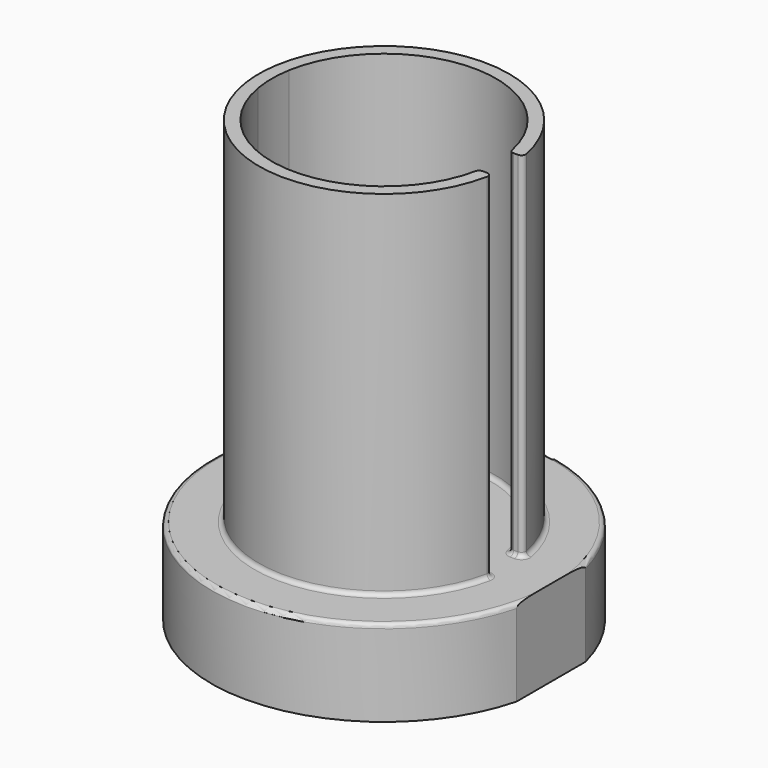
from build123d import *

# Parameters (mm, degrees)
F0_W     = 38.7298334621
F0_H     = 10
F1_DEPTH = 10
F3_DEPTH = 41
F4_F1_R  = 0.5
F4_F2_R  = 0.5


with BuildPart() as f1:
    # F0 (on Top) → F1 (new body)
    with BuildSketch(Plane.XY):
        with BuildLine():
            Line((-19.364916731, 5), (19.364916731, 5))
            ThreePointArc((19.364916731, 5), (0, 20), (-19.364916731, 5))
        make_face()
        Rectangle(F0_W, F0_H)
        with BuildLine():
            ThreePointArc((-19.364916731, -5), (0, -20), (19.364916731, -5))
            Line((19.364916731, -5), (-19.364916731, -5))
        make_face()
        with BuildLine():
            Line((-19.364916731, -5), (-19.364916731, 5))
            ThreePointArc((-19.364916731, 5), (-20, 0), (-19.364916731, -5))
        make_face()
    extrude(amount=-F1_DEPTH)

    # F2 (on face) → F3 (join)
    with BuildSketch(Plane.XY):
        with BuildLine():
            ThreePointArc((-12.8038080273, 2.25), (0, 13), (12.8038080273, 2.25))
            Line((12.8038080273, 2.25), (14.3243673508, 2.25))
            ThreePointArc((14.3243673508, 2.25), (0, 14.5), (-14.3243673508, 2.25))
            Line((-14.3243673508, 2.25), (-12.8038080273, 2.25))
        make_face()
        with BuildLine():
            Line((14.3243673508, -2.25), (12.8038080273, -2.25))
            ThreePointArc((12.8038080273, -2.25), (0, -13), (-12.8038080273, -2.25))
            Line((-12.8038080273, -2.25), (-14.3243673508, -2.25))
            ThreePointArc((-14.3243673508, -2.25), (0, -14.5), (14.3243673508, -2.25))
        make_face()
        with BuildLine():
            ThreePointArc((-12.8038080273, -2.25), (-13, 0), (-12.8038080273, 2.25))
            Line((-12.8038080273, 2.25), (-14.3243673508, 2.25))
            ThreePointArc((-14.3243673508, 2.25), (-14.5, 0), (-14.3243673508, -2.25))
            Line((-14.3243673508, -2.25), (-12.8038080273, -2.25))
        make_face()
    extrude(amount=F3_DEPTH)

    # F4: fillet of radius 0.5 on 7 edges, made by hand

    # F4_f1
    f4_f1_edges = [f1.edges().sort_by_distance(p)[0] for p in [
        (-20, 0, 0),
        (12.8038080273, 2.25, 20.5),
        (12.8038080273, -2.25, 20.5),
        (14.3243673508, 2.25, 20.5),
        (14.3243673508, -2.25, 20.5),
    ]]
    fillet(f4_f1_edges, radius=F4_F1_R)

    # F4_f2
    f4_f2_edges = [f1.edges().sort_by_distance(p)[0] for p in [
        (-14.5, 0, 0),
        (-13, 0, 0),
        (12.9014449798, -2.3621044432, 0),
        (12.9014449798, 2.3621044432, 0),
        (14.1139754816, 2.4330671545, 0),
        (14.1139754816, -2.4330671545, 0),
    ]]
    fillet(f4_f2_edges, radius=F4_F2_R)


solid = f1.part
